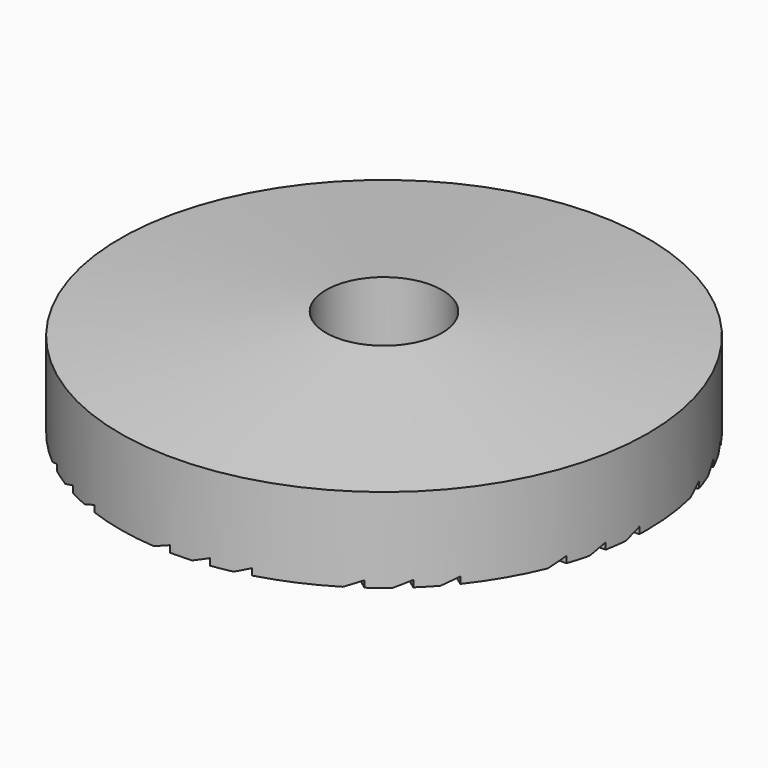
from build123d import *

# Parameters (mm, degrees)
F3_DEPTH         = 15.875
F3_COPIES_COUNT  = 4
F3_COPIES_ANGLE  = 108
F3_COPIES1_COUNT = 3
F3_COPIES1_ANGLE = 144
F3_COPIES2_COUNT = 2
F3_COPIES2_ANGLE = 108
F3_COPIES3_COUNT = 2
F3_COPIES4_COUNT = 2
F3_COPIES4_ANGLE = 36
F3_COPIES5_COUNT = 2
F3_COPIES5_ANGLE = 216
F4_DEPTH         = 15.875
F5_SIZE2         = 15.87499
F5_SIZE          = 38.09999
F7_DEPTH         = 38.1


# Not quite as in the source:
# - a fillet or chamfer is up to 0.001 mm smaller than in the source, because OpenCascade refuses the exact size
# - a pattern or mirror of a feature is missing from the dataset's text; its kind, count and spacing are read off the source's solid


with BuildPart() as f1:
    # F0 (on Front) → F1 (revolve)
    with BuildSketch(Plane.XZ):
        Polygon((139.7, 255.2581277271), (139.7, 0), (635, 0), (635, 203.2), align=None)
    revolve(axis=Axis((0, 0, 127.6290638635), (0, 0, 1)))

    # F2 (on face) → F3 (cut)
    with BuildSketch(Plane(origin=(0, 0, 0), x_dir=(1, 0, 0), z_dir=(0, 0, -1))):
        with BuildLine():
            Line((-150.2684264907, -25.4), (-634.4917966373, -25.4))
            ThreePointArc((-634.4917966373, -25.4), (-633.4409277083, -44.4701147299), (-631.8170225627, -63.5))
            Line((-631.8170225627, -63.5), (-138.5406438559, -63.5))
            ThreePointArc((-138.5406438559, -63.5), (-145.6556633936, -44.8351170555), (-150.2684264907, -25.4))
        make_face()
        with BuildLine():
            Line((-207.5208657794, -114.3), (-624.6282974698, -114.3))
            ThreePointArc((-624.6282974698, -114.3), (-620.8268829998, -133.4128230149), (-616.4407838552, -152.4))
            Line((-616.4407838552, -152.4), (-261.9333048363, -152.4))
            Line((-261.9333048363, -152.4), (-207.5208657794, -114.3))
        make_face()
        with BuildLine():
            ThreePointArc((-601.6101395422, -203.2), (-594.7934234718, -222.3640784721), (-587.3664188562, -241.3))
            Line((-587.3664188562, -241.3), (-388.8956626356, -241.3))
            Line((-388.8956626356, -241.3), (-334.4832235788, -203.2))
            Line((-334.4832235788, -203.2), (-601.6101395422, -203.2))
        make_face()
    f3 = extrude(amount=-F3_DEPTH, mode=Mode.SUBTRACT)

    # F3_copies: F3 ×4 about axis
    f3_copies_axis = Axis((0, 0, 0), (0, 0, -1))
    for i in range(1, F3_COPIES_COUNT):
        add(f3.rotate(f3_copies_axis, i * F3_COPIES_ANGLE / (F3_COPIES_COUNT - 1)), mode=Mode.SUBTRACT)

    # F3_copies1: F3 ×3 about axis
    f3_copies1_axis = Axis((0, 0, 0), (0, 0, 1))
    for i in range(1, F3_COPIES1_COUNT):
        add(f3.rotate(f3_copies1_axis, i * F3_COPIES1_ANGLE / (F3_COPIES1_COUNT - 1)), mode=Mode.SUBTRACT)

    # F3_copies2: F3 ×2 about axis
    f3_copies2_axis = Axis((0, 0, 0), (0, 0, 1))
    for i in range(1, F3_COPIES2_COUNT):
        add(f3.rotate(f3_copies2_axis, i * F3_COPIES2_ANGLE / (F3_COPIES2_COUNT - 1)), mode=Mode.SUBTRACT)

    # F3_copies3: F3 ×2 about axis
    f3_copies3_axis = Axis((0, 0, 0), (0, 0, 1))
    for i in range(1, F3_COPIES3_COUNT):
        add(f3.rotate(f3_copies3_axis, i * 360 / F3_COPIES3_COUNT), mode=Mode.SUBTRACT)

    # F3_copies4: F3 ×2 about axis
    f3_copies4_axis = Axis((0, 0, 0), (0, 0, 1))
    for i in range(1, F3_COPIES4_COUNT):
        add(f3.rotate(f3_copies4_axis, i * F3_COPIES4_ANGLE / (F3_COPIES4_COUNT - 1)), mode=Mode.SUBTRACT)

    # F3_copies5: F3 ×2 about axis
    f3_copies5_axis = Axis((0, 0, 0), (0, 0, 1))
    for i in range(1, F3_COPIES5_COUNT):
        add(f3.rotate(f3_copies5_axis, i * F3_COPIES5_ANGLE / (F3_COPIES5_COUNT - 1)), mode=Mode.SUBTRACT)

    # F2 (on face) → F4 (cut)
    with BuildSketch(Plane(origin=(0, 0, 0), x_dir=(1, 0, 0), z_dir=(0, 0, -1))):
        with BuildLine():
            ThreePointArc((152.4, 0), (-12.7446420666, 151.8661716729), (-150.2684264907, -25.4))
            Line((-150.2684264907, -25.4), (-137.3715035952, -25.4))
            ThreePointArc((-137.3715035952, -25.4), (-12.7532534624, 139.116657975), (139.7, 0))
            ThreePointArc((139.7, 0), (32.6546258056, -135.8299135445), (-124.4340789334, -63.5))
            Line((-124.4340789334, -63.5), (-138.5406438559, -63.5))
            ThreePointArc((-138.5406438559, -63.5), (32.4974297166, -148.8948523684), (152.4, 0))
        make_face()
        with BuildLine():
            Line((-37.1751710773, -25.4), (-137.3715035952, -25.4))
            ThreePointArc((-137.3715035952, -25.4), (-132.2816815012, -44.9182227968), (-124.4340789334, -63.5))
            Line((-124.4340789334, -63.5), (-37.1751710773, -63.5))
            Line((-37.1751710773, -63.5), (-37.1751710773, -25.4))
        make_face()
        with BuildLine():
            Line((-137.3715035952, -25.4), (-150.2684264907, -25.4))
            ThreePointArc((-150.2684264907, -25.4), (-145.6556633936, -44.8351170555), (-138.5406438559, -63.5))
            Line((-138.5406438559, -63.5), (-124.4340789334, -63.5))
            ThreePointArc((-124.4340789334, -63.5), (-132.2816815012, -44.9182227968), (-137.3715035952, -25.4))
        make_face()
    extrude(amount=-F4_DEPTH, mode=Mode.SUBTRACT)

    # F5 (size 38.1 and 15.875 in the source; OpenCascade refuses exactly that, so slightly less here)
    f5_edges = [f1.edges().sort_by_distance(p)[0] for p in [
        (-385.178833, 63.5, 15.875),
        (-439.187044, 152.4, 15.875),
        (-488.131041, 241.3, 15.875),
        (-274.291858, 277.775017, 15.875),
        (-58.634717, 385.949418, 15.875),
        (179.418894, 346.70426, 15.875),
        (348.940585, 175.029859, 15.875),
        (385.178833, -63.5, 15.875),
        (274.291858, -277.775017, 15.875),
        (58.634717, -385.949418, 15.875),
        (-179.418894, -346.70426, 15.875),
        (-348.940585, -175.029859, 15.875),
        (-444.888255, -134.853478, 15.875),
        (-536.738889, -91.700426, 15.875),
        (-280.657273, -370.59751, 15.875),
        (-380.330724, -389.674406, 15.875),
        (-9.224753, -464.78589, 15.875),
        (-78.64915, -538.806008, 15.875),
        (265.73131, -381.441858, 15.875),
        (253.073726, -482.132028, 15.875),
        (439.187044, -152.4, 15.875),
        (488.131041, -241.3, 15.875),
        (444.888255, 134.853478, 15.875),
        (536.738889, 91.700426, 15.875),
        (280.657273, 370.59751, 15.875),
        (380.330724, 389.674406, 15.875),
        (9.224753, 464.78589, 15.875),
        (78.64915, 538.806008, 15.875),
        (-265.73131, 381.441858, 15.875),
        (-253.073726, 482.132028, 15.875),
    ]]
    chamfer(f5_edges, length=F5_SIZE, length2=F5_SIZE2)

    # F6 (on face) → F7 (cut)
    with BuildSketch(Plane(origin=(0, 0, 0), x_dir=(1, 0, 0), z_dir=(0, 0, -1))):
        with BuildLine():
            Line((147.5606654905, 38.1), (-147.5606654905, 38.1))
            ThreePointArc((-147.5606654905, 38.1), (-152.2616317645, 6.4927261153), (-150.2684264907, -25.4))
            Line((-150.2684264907, -25.4), (-254, -25.4))
            Line((-254, -25.4), (-254, -38.1))
            Line((-254, -38.1), (147.5606654905, -38.1))
            ThreePointArc((147.5606654905, -38.1), (151.1853257111, -19.2030541744), (152.4, 0))
            ThreePointArc((152.4, 0), (151.1853257111, 19.2030541744), (147.5606654905, 38.1))
        make_face()
        with BuildLine():
            Line((-147.5606654905, 38.1), (-254, 38.1))
            Line((-254, 38.1), (-254, -25.4))
            Line((-254, -25.4), (-150.2684264907, -25.4))
            ThreePointArc((-150.2684264907, -25.4), (-152.2616317645, 6.4927261153), (-147.5606654905, 38.1))
        make_face()
        with BuildLine():
            Line((254, 38.1), (147.5606654905, 38.1))
            ThreePointArc((147.5606654905, 38.1), (151.1853257111, 19.2030541744), (152.4, 0))
            ThreePointArc((152.4, 0), (151.1853257111, -19.2030541744), (147.5606654905, -38.1))
            Line((147.5606654905, -38.1), (254, -38.1))
            Line((254, -38.1), (254, 38.1))
        make_face()
    extrude(amount=-F7_DEPTH, mode=Mode.SUBTRACT)


solid = f1.part
